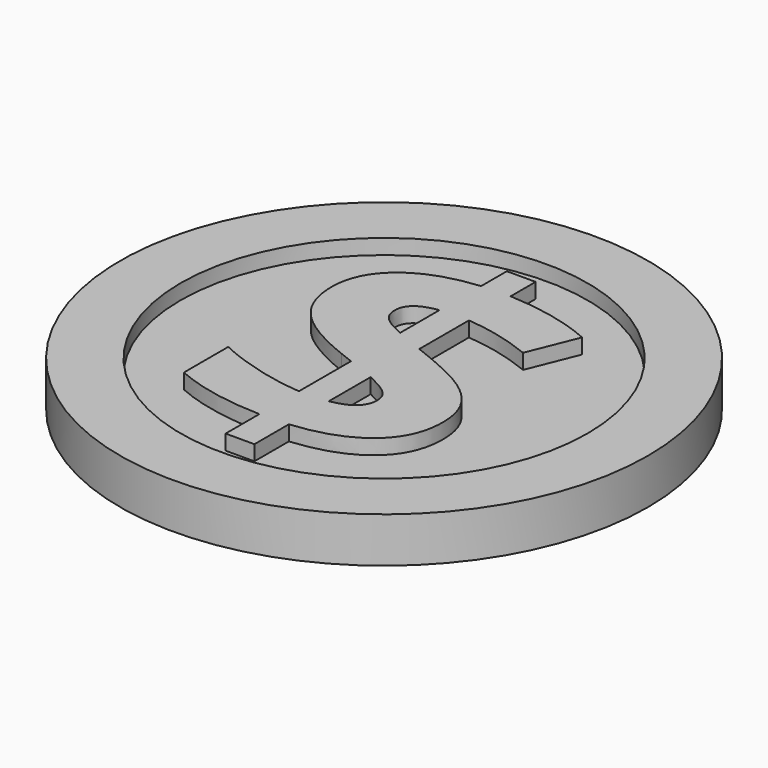
from build123d import *

# Parameters (mm, degrees)
F0_R         = 20.0025
F1_DEPTH     = 2.286
F2_TEXT_SIZE = 32.6100141845
F3_DEPTH     = 1.143
F4_R         = 20.0025
F4_R_2       = 15.4234662174
F5_DEPTH     = 1.143


# Not quite as in the source:
# - a feature of the source that left no trace in its solid (it failed there, or was rolled back) is left out
# - Text() gives the source's letters only with a copy of the font that has no kerning and outlines rounded to 1/6400 em; it was checked with that copy


with BuildPart() as f1:
    # F0 (on Top) → F1 (new body)
    with BuildSketch(Plane.XY):
        Circle(F0_R)
    extrude(amount=F1_DEPTH)

    # F2 (on face) → F3 (join)
    with BuildSketch(Plane.XY.offset(2.286)):
        with Locations((-9.543960914, -11.4971324801)):
            Text('$', F2_TEXT_SIZE, font='Open Sans', font_style=FontStyle.BOLD, text_align=(TextAlign.LEFT, TextAlign.BOTTOM))
    extrude(amount=F3_DEPTH)

    # F4 (on face) → F5 (join, through all)
    with BuildSketch(Plane.XY.offset(2.286)):
        Circle(F4_R)
        Circle(F4_R_2, mode=Mode.SUBTRACT)
    extrude(amount=F5_DEPTH)


solid = f1.part
